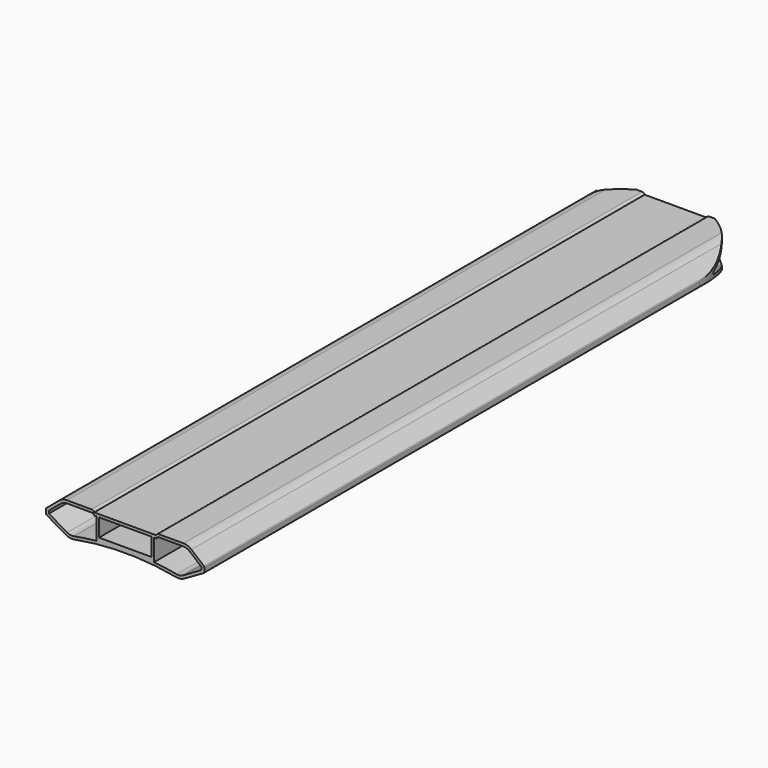
from build123d import *

# Parameters (mm, degrees)
F2_DEPTH       = 500
F1_W           = 38
F1_H           = 13
F3_DEPTH       = 600
F4_T1_DEPTH    = 509.3674969976
F5_R           = 9
F6_R           = 1
F8_DEPTH       = 500.001
F10_DEPTH      = 16.8433111076
F10_DEPTH_BACK = 25


# Not quite as in the source:
# - a fillet or chamfer that OpenCascade refuses, or shapes differently, is made with other operations: its cross-section is extruded or revolved along the edge and cut away or added
# - ends of sketch curves that miss each other by under 0.0002 mm in the source are joined


with BuildPart() as f2:
    # F0 (on Front) → F2 (new body)
    with BuildSketch(Plane.XZ):
        with BuildLine():
            Line((22.5, 5.3759940737), (0, 5.3759940737))
            Line((0, 5.3759940737), (-22.5, 5.3759940737))
            Line((-22.5, 5.3759940737), (-22.5, 6.6759940737))
            Line((-22.5, 6.6759940737), (-45.5824640741, 6.6759940737))
            Line((-45.5824640741, 6.6759940737), (-57.5, -3.3240059263))
            Line((-57.5, -3.3240059263), (-57.5, -7.3240059263))
            Line((-57.5, -7.3240059263), (-40.1794919243, -17.3240059263))
            ThreePointArc((-40.1794919243, -17.3240059263), (0, -13.2464610679), (40.1794919243, -17.3240059263))
            Line((40.1794919243, -17.3240059263), (57.5, -7.3240059263))
            Line((57.5, -7.3240059263), (57.5, -3.3240059263))
            Line((57.5, -3.3240059263), (45.5824640741, 6.6759940737))
            Line((45.5824640741, 6.6759940737), (22.5, 6.6759940737))
            Line((22.5, 6.6759940737), (22.5, 5.3759940737))
        make_face()
    extrude(amount=F2_DEPTH)

    # F1 (on face) → F3 (cut)
    with BuildSketch(Plane.XZ):
        with Locations((0, -3.1240059263)):
            Rectangle(F1_W, F1_H)
    extrude(amount=F3_DEPTH, mode=Mode.SUBTRACT)

    # F4: fillet of radius 2 on 2 edges, made by hand

    # F4_s2 → F4_t1 (cut)
    with BuildSketch(Plane.XZ.offset(-4.6837484988)):
        with BuildLine():
            ThreePointArc((-24.3734993995, 6.6759940737), (-23.2333239744, 6.3191617462), (-22.5, 5.3759940737))
            Line((-22.5, 5.3759940737), (-22.5, 6.6759940737))
            Line((-22.5, 6.6759940737), (-24.3734993995, 6.6759940737))
        make_face()
        with BuildLine():
            ThreePointArc((24.3734993995, 6.6759940737), (23.2333239744, 6.3191617462), (22.5, 5.3759940737))
            Line((22.5, 5.3759940737), (22.5, 6.6759940737))
            Line((22.5, 6.6759940737), (24.3734993995, 6.6759940737))
        make_face()
    extrude(amount=F4_T1_DEPTH, mode=Mode.SUBTRACT)

    # F5
    f5_edges = [f2.edges().sort_by_distance(p)[0] for p in [
        (-45.582464, -250, 6.675994),
        (-40.179492, -250, -17.324006),
        (40.179492, -250, -17.324006),
        (45.582464, -250, 6.675994),
    ]]
    fillet(f5_edges, radius=F5_R)

    # F6
    f6_edges = [f2.edges().sort_by_distance(p)[0] for p in [
        (57.5, -250, -3.324006),
        (57.5, -250, -7.324006),
        (-57.5, -250, -7.324006),
        (-57.5, -250, -3.324006),
    ]]
    fillet(f6_edges, radius=F6_R)

    # F7 (on face) → F8 (cut, through all)
    with BuildSketch(Plane.XZ.offset(500)):
        with BuildLine():
            ThreePointArc((-42.1022688854, -13.9044885758), (-39.7790672738, -14.7426835793), (-37.3093702039, -14.7218755322))
            ThreePointArc((-37.3093702039, -14.7218755322), (-29.1789784784, -13.3650277579), (-20.9999997169, -12.3410102235))
            Line((-20.9999997169, -12.3410102235), (-20.9999997169, 3.3759940737))
            Line((-20.9999997169, 3.3759940737), (-22.5, 3.3759940737))
            ThreePointArc((-22.5, 3.3759940737), (-23.2333240923, 4.3191614627), (-24.3734993995, 4.67599366))
            Line((-24.3734993995, 4.67599366), (-42.3067319657, 4.67599366))
            ThreePointArc((-42.3067319657, 4.67599366), (-44.7008728275, 4.2538420304), (-46.8062449676, 3.0383048586))
            Line((-46.8062449676, 3.0383048586), (-55.4999995863, -4.2566214356))
            Line((-55.4999995863, -4.2566214356), (-55.4999995863, -6.1693051491))
            Line((-55.4999995863, -6.1693051491), (-42.1022688854, -13.9044885758))
        make_face()
        with BuildLine():
            Line((20.9999997169, 3.3759940737), (20.9999997169, -12.3410102235))
            ThreePointArc((20.9999997169, -12.3410102235), (29.1789784784, -13.3650277579), (37.3093702039, -14.7218755322))
            ThreePointArc((37.3093702039, -14.7218755322), (39.7790673581, -14.7426840737), (42.1022691362, -13.9044890102))
            Line((42.1022691362, -13.9044890102), (55.5000000879, -6.1693054387))
            Line((55.5000000879, -6.1693054387), (55.5000000879, -4.2566212017))
            Line((55.5000000879, -4.2566212017), (46.8062452899, 3.0383052428))
            ThreePointArc((46.8062452899, 3.0383052428), (44.700872999, 4.2538425017), (42.3067319657, 4.6759941615))
            Line((42.3067319657, 4.6759941615), (24.3734993995, 4.6759941615))
            ThreePointArc((24.3734993995, 4.6759941615), (23.2333239494, 4.3191618064), (22.5, 3.3759940737))
            Line((22.5, 3.3759940737), (20.9999997169, 3.3759940737))
        make_face()
    extrude(amount=-F8_DEPTH, mode=Mode.SUBTRACT)

    # F9 (on Top) → F10 (cut, two sides)
    with BuildSketch(Plane.XY) as f10_sk:
        with BuildLine():
            ThreePointArc((-57.495400138, -49.2727015938), (0.3636564761, 7.498850023), (57.5, -50))
            Line((57.5, -50), (57.8162293472, 0))
            Line((57.8162293472, 0), (57.8162293472, 30))
            Line((57.8162293472, 30), (-57.1837706528, 30))
            Line((-57.1837706528, 30), (-57.1837706528, 0))
            Line((-57.1837706528, 0), (-57.495400138, -49.2727015938))
        make_face()
    extrude(amount=-F10_DEPTH, mode=Mode.SUBTRACT)
    extrude(f10_sk.sketch, amount=F10_DEPTH_BACK, mode=Mode.SUBTRACT)


solid = f2.part
